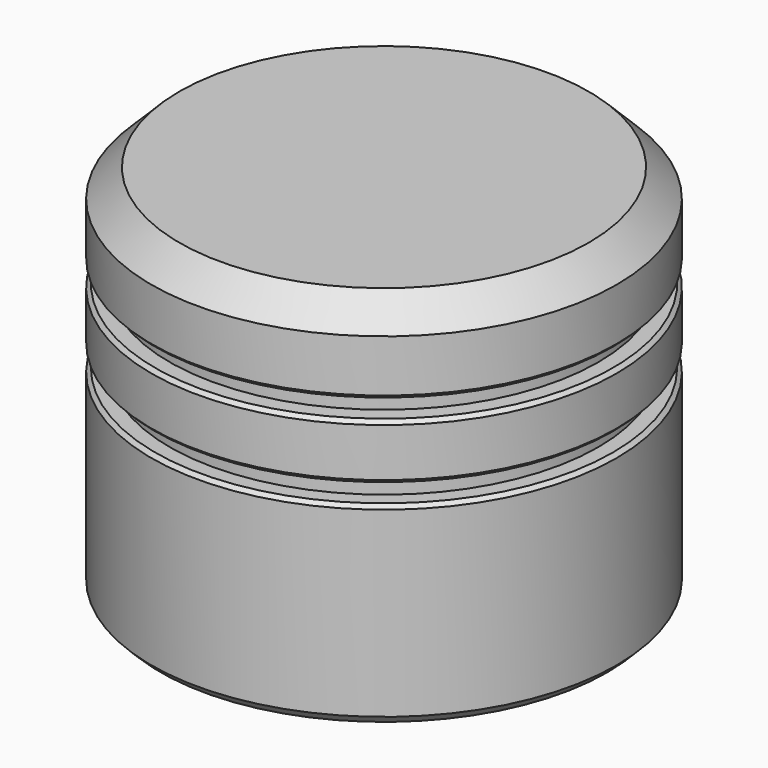
from build123d import *

# Parameters (mm, degrees)
F0_R        = 12.5
F1_DEPTH    = 20
F2_R        = 3.625
F3_DEPTH    = 19.5
F4_SIZE     = 1.5
F5_SIZE     = 0.5
F6_W        = 1
F6_H        = 1
F8_T4_ANGLE = 270
F8_T6_ANGLE = 90


# Not quite as in the source:
# - a fillet or chamfer that OpenCascade refuses, or shapes differently, is made with other operations: its cross-section is extruded or revolved along the edge and cut away or added


with BuildPart() as f1:
    # F0 (on Top) → F1 (new body)
    with BuildSketch(Plane.XY):
        Circle(F0_R)
    extrude(amount=F1_DEPTH)

    # F2 (on Top) → F3 (cut)
    with BuildSketch(Plane.XY):
        Circle(F2_R)
    extrude(amount=F3_DEPTH, mode=Mode.SUBTRACT)

    # F4
    f4_edges = [f1.edges().sort_by_distance(p)[0] for p in [
        (-12.5, 0, 20),
    ]]
    chamfer(f4_edges, length=F4_SIZE)

    # F5
    f5_edges = [f1.edges().sort_by_distance(p)[0] for p in [
        (-12.5, 0, 0),
        (-3.625, 0, 0),
    ]]
    chamfer(f5_edges, length=F5_SIZE)

    # F6 (on Right) → F7 (revolve, cut)
    with BuildSketch(Plane.YZ):
        Polygon((12.5177614391, 14.5), (12.5177614391, 15.5), (11.5177614391, 15.5), (11.5177614391, 14.5179004222), align=None)
        with Locations((12.0177614391, 11)):
            Rectangle(F6_W, F6_H)
    revolve(axis=Axis((0, 0, 0), (0, 0, -1)), mode=Mode.SUBTRACT)

    # F8: chamfer of 0.2 on 5 edges, made by hand

    # F8_s1 → F8_t2 (revolve, cut)
    with BuildSketch(Plane.XZ):
        Polygon((12.3, 15.5), (12.5, 15.7), (12.5, 15.5), align=None)
    revolve(axis=Axis((0, 0, 15.5), (0, 0, -1)), mode=Mode.SUBTRACT)

    # F8_s3 → F8_t4 (revolve, cut)
    with BuildSketch(Plane.XZ):
        Polygon((12.5, 14.3038659818), (12.303579511, 14.5038339469), (12.5, 14.5003179373), align=None)
    revolve(axis=Axis((0, 0, 14.5003179373), (0, 0, -1)), revolution_arc=F8_T4_ANGLE, mode=Mode.SUBTRACT)

    # F8_s5 → F8_t6 (revolve, cut)
    with BuildSketch(Plane.YZ):
        Polygon((12.5, 14.3038659818), (12.303579511, 14.5038339469), (12.5, 14.5003179373), align=None)
    revolve(axis=Axis((0, 0, 14.5003179373), (0, 0, -1)), revolution_arc=F8_T6_ANGLE, mode=Mode.SUBTRACT)

    # F8_s7 → F8_t8 (revolve, cut)
    with BuildSketch(Plane.XZ):
        Polygon((12.3, 11.5), (12.5, 11.7), (12.5, 11.5), align=None)
    revolve(axis=Axis((0, 0, 11.5), (0, 0, -1)), mode=Mode.SUBTRACT)

    # F8_s9 → F8_t10 (revolve, cut)
    with BuildSketch(Plane.XZ):
        Polygon((12.5, 10.3), (12.3, 10.5), (12.5, 10.5), align=None)
    revolve(axis=Axis((0, 0, 10.5), (0, 0, -1)), mode=Mode.SUBTRACT)


solid = f1.part
